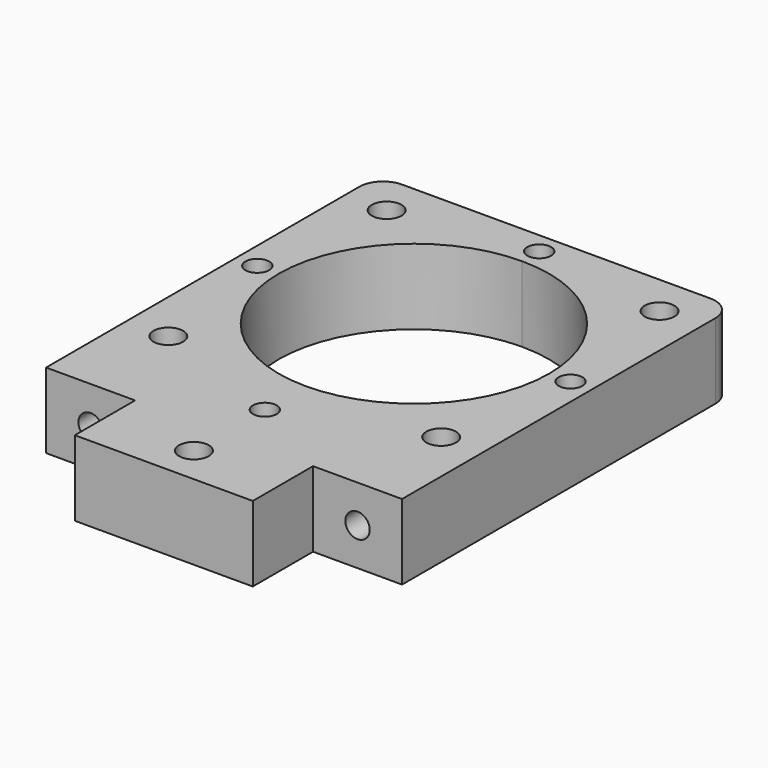
from build123d import *

# Parameters (mm, degrees)
F0_W           = 15
F0_H           = 6.35
F1_DEPTH       = 6.35
F2_R           = 2
F5_D           = 2.05
F5_DEPTH       = 6
F5_TIP         = 0.6158821345
F5_ON_F3_D     = 2.05
F5_ON_F3_DEPTH = 6
F5_ON_F3_TIP   = 0.6158821345
F6_D           = 2.5
F6_CSINK_D     = 4.7
F6_CSINK_ANGLE = 90
F7_D           = 2
F7_DEPTH       = 8
F7_TIP         = 0.600860619


# Not quite as in the source:
# - a length typed as a fraction of an inch, garbled in the dataset ("3 / 203.2 mm" for 3/8 in), is restored


with BuildPart() as f1:
    # F0 (on Top) → F1 (new body)
    with BuildSketch(Plane.XY):
        Polygon((15, 15), (-15, 15), (-15, -20), (-7.5, -20), (7.5, -20), (15, -20), align=None)
        with BuildLine():
            ThreePointArc((0, 11.4), (8.0610173055, 8.0610173055), (11.4, 0))
            ThreePointArc((11.4, 0), (-8.0610173055, -8.0610173055), (0, 11.4))
        make_face(mode=Mode.SUBTRACT)
        with Locations((0, -23.175)):
            Rectangle(F0_W, F0_H)
    extrude(amount=F1_DEPTH)

    # F2
    f2_edges = [f1.edges().sort_by_distance(p)[0] for p in [
        (15, 15, 3.175),
        (-15, 15, 3.175),
    ]]
    fillet(f2_edges, radius=F2_R)

    # F5
    with Locations(Plane.XZ.offset(20)):
        with Locations((-11.25, 3.175)):
            Hole(F5_D / 2, depth=F5_DEPTH)
            with Locations((0, 0, -(F5_DEPTH + F5_TIP / 2))):  # 118° drill point
                Cone(0, F5_D / 2, F5_TIP, mode=Mode.SUBTRACT)

    # F5 on F3
    with Locations(Plane.XZ.offset(20)):
        with Locations((11.25, 3.175)):
            Hole(F5_ON_F3_D / 2, depth=F5_ON_F3_DEPTH)
            with Locations((0, 0, -(F5_ON_F3_DEPTH + F5_ON_F3_TIP / 2))):  # 118° drill point
                Cone(0, F5_ON_F3_D / 2, F5_ON_F3_TIP, mode=Mode.SUBTRACT)

    # F6 (through all)
    with Locations(Plane(origin=(0, 0, 0), x_dir=(1, 0, 0), z_dir=(0, 0, -1))):
        with Locations((-11.5, -11.5), (11.5, -11.5), (-11.5, 11.5), (11.5, 11.5), (0, 23.175)):
            CounterSinkHole(F6_D / 2, F6_CSINK_D / 2, counter_sink_angle=F6_CSINK_ANGLE)

    # F7
    with Locations(Plane(origin=(0, 0, 0), x_dir=(1, 0, 0), z_dir=(0, 0, -1))):
        with Locations((13.2, 0), (0, -13.2), (-13.2, 0), (0, 15.7)):
            Hole(F7_D / 2, depth=F7_DEPTH)
            with Locations((0, 0, -(F7_DEPTH + F7_TIP / 2))):  # 118° drill point
                Cone(0, F7_D / 2, F7_TIP, mode=Mode.SUBTRACT)


solid = f1.part
